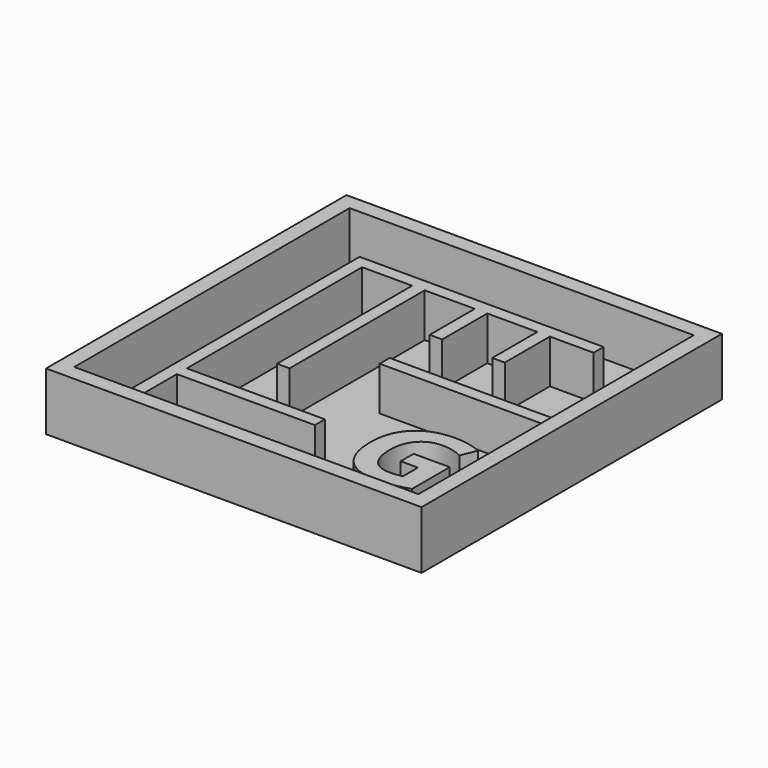
from build123d import *

# Parameters (mm, degrees)
F0_W         = 38.1
F0_H         = 38.1
F1_DEPTH     = 0.79375
F2_W         = 38.1
F2_H         = 38.1
F2_W_2       = 34.925
F2_H_2       = 34.925
F3_DEPTH     = 5.08
F4_W         = 14.0040102594
F4_H         = 1.27
F4_W_2       = 1.27
F4_H_2       = 17.145
F4_H_3       = 5.715
F4_W_3       = 17.145
F5_DEPTH     = 4.445
F6_R         = 1.27
F7_DEPTH     = 0.396875
F8_TEXT_SIZE = 12.9430309042
F9_DEPTH     = 4.445


# Not quite as in the source:
# - Text() gives the source's letters only with a copy of the font that has no kerning and outlines rounded to 1/6400 em; it was checked with that copy


with BuildPart() as f1:
    # F0 (on Top) → F1 (new body)
    with BuildSketch(Plane.XY):
        with Locations((-0.7093064487, -3.367246665)):
            Rectangle(F0_W, F0_H)
    extrude(amount=F1_DEPTH)

    # F2 (on face) → F3 (join)
    with BuildSketch(Plane.XY.offset(0.79375)):
        with Locations((-0.7093064487, -3.367246665)):
            Rectangle(F2_W, F2_H)
        with Locations((-0.7093064487, -3.367246665)):
            Rectangle(F2_W_2, F2_H_2, mode=Mode.SUBTRACT)
    extrude(amount=F3_DEPTH)

    # F4 (on face) → F5 (join)
    with BuildSketch(Plane.XY.offset(0.79375)):
        Polygon((-13.0918064487, -20.829746665), (-11.8218064487, -20.829746665), (-11.8218064487, -15.749746665), (-11.8218064487, -14.479746665), (-11.8218064487, 7.745253335), (-11.8218064487, 9.015253335), (-13.0918064487, 9.015253335), align=None)
        with Locations((-4.819801319, -15.114746665)):
            Rectangle(F4_W, F4_H)
        Polygon((11.6731935513, 9.015253335), (-11.8218064487, 9.015253335), (-11.8218064487, 7.745253335), (-6.7418064487, 7.745253335), (-5.4718064487, 7.745253335), (-0.3918064487, 7.745253335), (0.8781935513, 7.745253335), (5.9581935513, 7.745253335), (7.2281935513, 7.745253335), (11.6731935513, 7.745253335), align=None)
        with Locations((-6.1068064487, -0.827246665)):
            Rectangle(F4_W_2, F4_H_2)
        with Locations((6.5931935513, 4.887753335)):
            Rectangle(F4_W_2, F4_H_3)
        with Locations((0.2431935513, 4.887753335)):
            Rectangle(F4_W_2, F4_H_3)
        with Locations((8.1806935513, -3.684746665)):
            Rectangle(F4_W_3, F4_H)
    extrude(amount=F5_DEPTH)

    # F6 (on face) → F7 (cut)
    with BuildSketch(Plane.XY.offset(0.79375)):
        with Locations((-15.6318064487, -17.8101807833)):
            Circle(F6_R)
        with Locations((-9.3015274033, -18.289746665)):
            Circle(F6_R)
    extrude(amount=-F7_DEPTH, mode=Mode.SUBTRACT)

    # F8 (on face) → F9 (join)
    with BuildSketch(Plane.XY.offset(0.79375)):
        with Locations((6.6964239813, -19.8965370655)):
            Text('G', F8_TEXT_SIZE, font='Open Sans', font_style=FontStyle.BOLD, text_align=(TextAlign.LEFT, TextAlign.BOTTOM))
    extrude(amount=F9_DEPTH)


solid = f1.part
